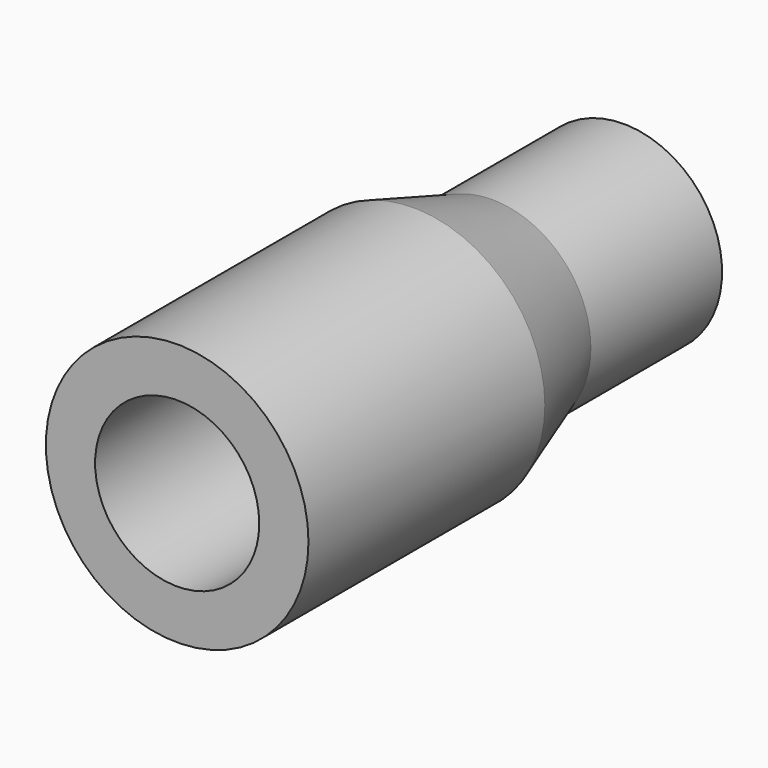
from build123d import *

# Parameters (mm, degrees)
F0_R     = 4
F0_R_2   = 2.5
F1_DEPTH = 12
F2_R     = 3
F2_R_2   = 2.5
F3_DEPTH = 5
F4_SIZE2 = 0.99999
F4_SIZE  = 2.99999


# Not quite as in the source:
# - a fillet or chamfer is up to 0.001 mm smaller than in the source, because OpenCascade refuses the exact size


with BuildPart() as f1:
    # F0 (on Front) → F1 (new body)
    with BuildSketch(Plane.XZ):
        Circle(F0_R)
        Circle(F0_R_2, mode=Mode.SUBTRACT)
    extrude(amount=F1_DEPTH)

    # F2 (on face) → F3 (join)
    with BuildSketch(Plane(origin=(0, 0, 0), x_dir=(-1, 0, 0), z_dir=(0, 1, 0))):
        Circle(F2_R)
        Circle(F2_R_2, mode=Mode.SUBTRACT)
    extrude(amount=F3_DEPTH)

    # F4 (size 3 and 1 in the source; OpenCascade refuses exactly that, so slightly less here)
    f4_edges = [f1.edges().sort_by_distance(p)[0] for p in [
        (-4, 0, 0),
    ]]
    f4_side = f1.faces().sort_by_distance((-4, -6, 0))[0]
    chamfer(f4_edges, length=F4_SIZE, length2=F4_SIZE2, reference=f4_side)


solid = f1.part
